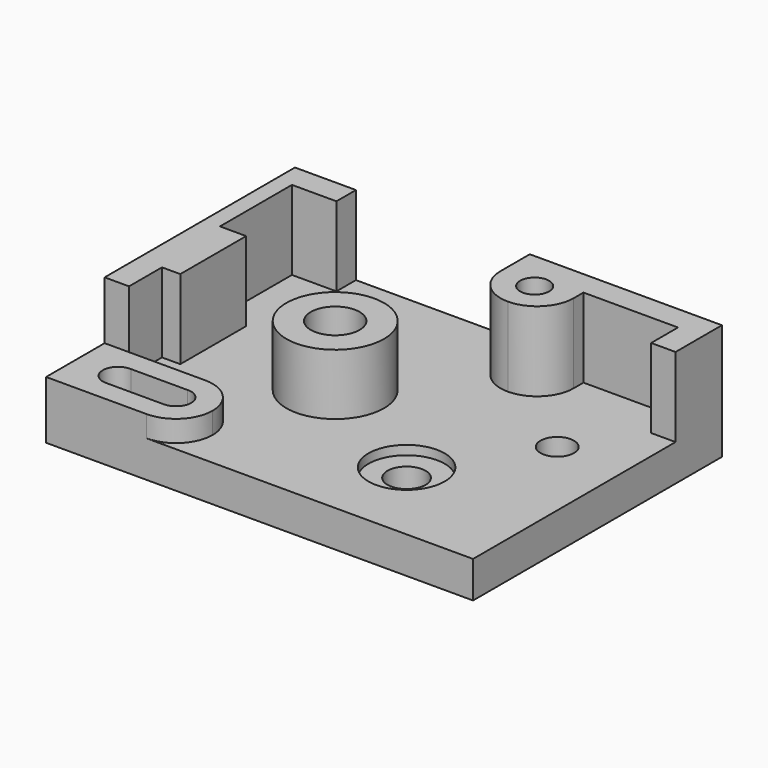
from build123d import *

# Parameters (mm, degrees)
F0_W      = 140
F0_H      = 38
F1_DEPTH  = 102
F2_R      = 4.75
F3_DEPTH  = 40
F4_R      = 8
F5_DEPTH  = 40
F6_R      = 6.25
F7_DEPTH  = 40
F8_R      = 5.5
F9_DEPTH  = 40
F10_W     = 140
F10_H     = 26
F11_DEPTH = 102
F12_R     = 16
F13_DEPTH = 26
F14_R     = 8
F15_DEPTH = 26
F16_W     = 45
F16_H     = 24
F17_DEPTH = 7
F18_R     = 12
F19_R     = 11.99999
F20_W     = 20
F20_H     = 78
F21_DEPTH = 26
F22_W     = 63
F22_H     = 24
F23_DEPTH = 26
F24_R     = 4.75
F25_DEPTH = 38
F26_R     = 12
F27_R     = 5
F28_DEPTH = 40
F30_DEPTH = 40
F31_W     = 19
F31_H     = 5
F32_DEPTH = 40
F33_W     = 31
F33_H     = 16
F34_DEPTH = 26
F35_R     = 11.99999
F36_W     = 8
F36_H     = 5
F37_DEPTH = 26
F38_R     = 16
F39_DEPTH = 6
F40_W     = 6
F40_H     = 74.1499609053
F41_DEPTH = 26
F42_W     = 6
F42_H     = 4
F43_DEPTH = 26
F44_W     = 6
F44_H     = 13.5
F45_DEPTH = 26
F46_W     = 8.5837110281
F46_H     = 29.5
F47_DEPTH = 26
F48_W     = 6
F48_H     = 0.1499609053
F49_DEPTH = 26
F50_R     = 12.5
F51_DEPTH = 3


# Not quite as in the source:
# - a fillet or chamfer is up to 0.001 mm smaller than in the source, because OpenCascade refuses the exact size


with BuildPart() as f1:
    # F0 (on Front) → F1 (new body)
    with BuildSketch(Plane.XZ):
        with Locations((70, 19)):
            Rectangle(F0_W, F0_H)
    extrude(amount=F1_DEPTH)

    # F2 (on face) → F3 (cut)
    with BuildSketch(Plane.XY.offset(38)):
        with Locations((35, -13)):
            Circle(F2_R)
        with Locations((89, -13)):
            Circle(F2_R)
    extrude(amount=-F3_DEPTH, mode=Mode.SUBTRACT)

    # F4 (on face) → F5 (cut)
    with BuildSketch(Plane.XY.offset(38)):
        with Locations((54, -51)):
            Circle(F4_R)
    extrude(amount=-F5_DEPTH, mode=Mode.SUBTRACT)

    # F6 (on face) → F7 (cut)
    with BuildSketch(Plane.XY.offset(38)):
        with Locations((95, -73)):
            Circle(F6_R)
    extrude(amount=-F7_DEPTH, mode=Mode.SUBTRACT)

    # F8 (on face) → F9 (cut)
    with BuildSketch(Plane.XY.offset(38)):
        with Locations((118, -40)):
            Circle(F8_R)
    extrude(amount=-F9_DEPTH, mode=Mode.SUBTRACT)

    # F10 (on face) → F11 (cut)
    with BuildSketch(Plane.XZ.offset(102)):
        with Locations((70, 25)):
            Rectangle(F10_W, F10_H)
    extrude(amount=-F11_DEPTH, mode=Mode.SUBTRACT)

    # F12 (on face) → F13 (join)
    with BuildSketch(Plane.XY.offset(12)):
        with Locations((54, -51)):
            Circle(F12_R)
    extrude(amount=F13_DEPTH)

    # F14 (on face) → F15 (cut)
    with BuildSketch(Plane.XY.offset(38)):
        with Locations((54, -51)):
            Circle(F14_R)
    extrude(amount=-F15_DEPTH, mode=Mode.SUBTRACT)

    # F16 (on face) → F17 (join)
    with BuildSketch(Plane.XY.offset(12)):
        with Locations((22.5, -90)):
            Rectangle(F16_W, F16_H)
    extrude(amount=F17_DEPTH)

    # F18
    f18_edges = [f1.edges().sort_by_distance(p)[0] for p in [
        (45, -78, 15.5),
    ]]
    fillet(f18_edges, radius=F18_R)

    # F19 (radius 12 in the source; OpenCascade refuses exactly that, so slightly less here)
    f19_edges = [f1.edges().sort_by_distance(p)[0] for p in [
        (45, -102, 15.5),
    ]]
    fillet(f19_edges, radius=F19_R)

    # F20 (on face) → F21 (join)
    with BuildSketch(Plane.XY.offset(12)):
        with Locations((10, -39)):
            Rectangle(F20_W, F20_H)
    extrude(amount=F21_DEPTH)

    # F22 (on face) → F23 (join)
    with BuildSketch(Plane.XY.offset(12)):
        with Locations((108.5, -12)):
            Rectangle(F22_W, F22_H)
    extrude(amount=F23_DEPTH)

    # F24 (on face) → F25 (cut)
    with BuildSketch(Plane(origin=(0, 0, 0), x_dir=(1, 0, 0), z_dir=(0, 0, -1))):
        with Locations((89, 13)):
            Circle(F24_R)
    extrude(amount=-F25_DEPTH, mode=Mode.SUBTRACT)

    # F26
    f26_edges = [f1.edges().sort_by_distance(p)[0] for p in [
        (77, -24, 25),
    ]]
    fillet(f26_edges, radius=F26_R)

    # F27 (on face) → F28 (cut)
    with BuildSketch(Plane.XY.offset(19)):
        with Locations((14, -90)):
            Circle(F27_R)
        with Locations((33, -90)):
            Circle(F27_R)
    extrude(amount=-F28_DEPTH, mode=Mode.SUBTRACT)

    # F29 (on face) → F30 (cut)
    with BuildSketch(Plane.XY.offset(19)):
        with BuildLine():
            ThreePointArc((14.2498681067, -85.00624731), (17.6227986788, -86.5539399696), (19, -90))
            Line((19, -90), (28, -90))
            ThreePointArc((28, -90), (29.3772013212, -86.5539399696), (32.7501318933, -85.00624731))
            Line((32.7501318933, -85.00624731), (14.2498681067, -85.00624731))
        make_face()
    extrude(amount=-F30_DEPTH, mode=Mode.SUBTRACT)

    # F31 (on face) → F32 (cut)
    with BuildSketch(Plane.XY.offset(19)):
        with Locations((23.5, -92.5)):
            Rectangle(F31_W, F31_H)
    extrude(amount=-F32_DEPTH, mode=Mode.SUBTRACT)

    # F33 (on face) → F34 (cut)
    with BuildSketch(Plane.XY.offset(38)):
        with Locations((116.5, -16)):
            Rectangle(F33_W, F33_H)
    extrude(amount=-F34_DEPTH, mode=Mode.SUBTRACT)

    # F35 (radius 12 in the source; OpenCascade refuses exactly that, so slightly less here)
    f35_edges = [f1.edges().sort_by_distance(p)[0] for p in [
        (101, -24, 25),
    ]]
    fillet(f35_edges, radius=F35_R)

    # F36 (on face) → F37 (cut)
    with BuildSketch(Plane.XY.offset(38)):
        with Locations((136, -21.5)):
            Rectangle(F36_W, F36_H)
    extrude(amount=-F37_DEPTH, mode=Mode.SUBTRACT)

    # F38 (on face) → F39 (cut)
    with BuildSketch(Plane.XY.offset(38)):
        with Locations((54, -51)):
            Circle(F38_R)
    extrude(amount=-F39_DEPTH, mode=Mode.SUBTRACT)

    # F40 (on face) → F41 (cut)
    with BuildSketch(Plane.XY.offset(38)):
        with Locations((17, -40.9250195473)):
            Rectangle(F40_W, F40_H)
    extrude(amount=-F41_DEPTH, mode=Mode.SUBTRACT)

    # F42 (on face) → F43 (join)
    with BuildSketch(Plane.XY.offset(12)):
        with Locations((17, -5.8500390947)):
            Rectangle(F42_W, F42_H)
    extrude(amount=F43_DEPTH)

    # F44 (on face) → F45 (cut)
    with BuildSketch(Plane.XY.offset(38)):
        with Locations((11, -71.25)):
            Rectangle(F44_W, F44_H)
    extrude(amount=-F45_DEPTH, mode=Mode.SUBTRACT)

    # F46 (on face) → F47 (cut)
    with BuildSketch(Plane.XY.offset(38)):
        with Locations((9.708144486, -22.75)):
            Rectangle(F46_W, F46_H)
    extrude(amount=-F47_DEPTH, mode=Mode.SUBTRACT)

    # F48 (on face) → F49 (join)
    with BuildSketch(Plane.XY.offset(38)):
        with Locations((17, -7.9250195473)):
            Rectangle(F48_W, F48_H)
    extrude(amount=-F49_DEPTH)

    # F50 (on face) → F51 (cut)
    with BuildSketch(Plane.XY.offset(12)):
        with Locations((95, -73)):
            Circle(F50_R)
    extrude(amount=-F51_DEPTH, mode=Mode.SUBTRACT)


solid = f1.part
